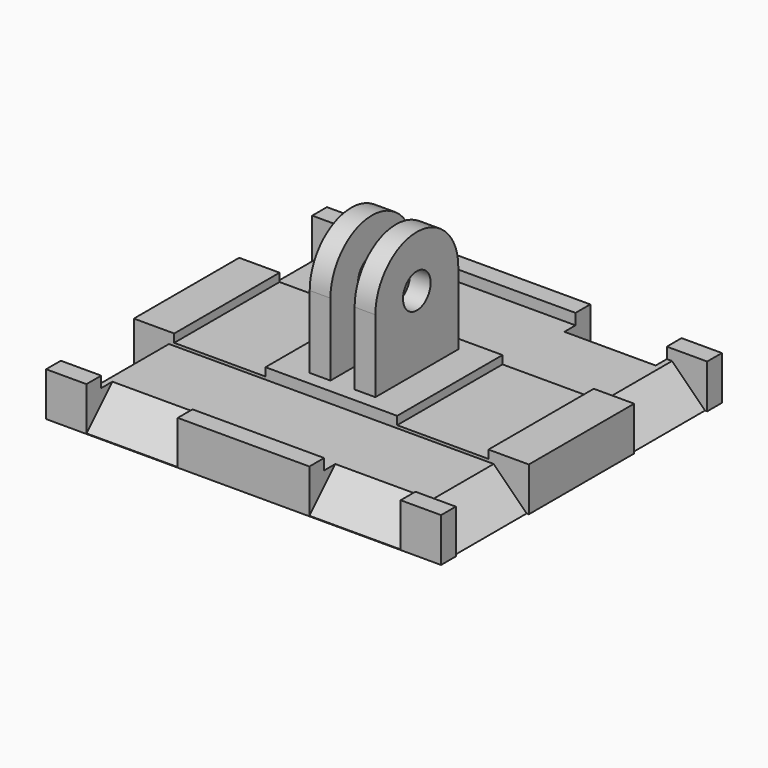
from build123d import *

# Parameters (mm, degrees)
F0_W         = 57.15
F0_H         = 50.8
F1_DEPTH     = 6.35
F2_W         = 13.208
F2_H         = 1.190625
F3_DEPTH     = 50.801
F4_SIZE      = 5.08
F5_W         = 3
F5_H         = 15
F6_DEPTH     = 18
F8_D         = 5
F9_W         = 13.208
F9_H         = 1.5875
F10_DEPTH    = 57.151
F11_T1_DEPTH = 13.208
F11_T3_DEPTH = 13.208
F13_DEPTH    = 33.326


# Not quite as in the source:
# - a fillet or chamfer that OpenCascade refuses, or shapes differently, is made with other operations: its cross-section is extruded or revolved along the edge and cut away or added


with BuildPart() as f1:
    # F0 (on Top) → F1 (new body)
    with BuildSketch(Plane.XY):
        Rectangle(F0_W, F0_H)
    extrude(amount=F1_DEPTH)

    # F2 (on face) → F3 (cut, through all)
    with BuildSketch(Plane.XZ.offset(25.4)):
        with Locations((-16.129, 5.7546875)):
            Rectangle(F2_W, F2_H)
        with Locations((16.129, 5.7546875)):
            Rectangle(F2_W, F2_H)
    extrude(amount=-F3_DEPTH, mode=Mode.SUBTRACT)

    # F4
    f4_edges = [f1.edges().sort_by_distance(p)[0] for p in [
        (-16.129, -25.4, 5.159375),
        (16.129, -25.4, 5.159375),
        (-16.129, 25.4, 5.159375),
        (16.129, 25.4, 5.159375),
    ]]
    chamfer(f4_edges, length=F4_SIZE)

    # F5 (on face) → F6 (join)
    with BuildSketch(Plane.XY.offset(6.35)):
        with Locations((-3.25, 0)):
            Rectangle(F5_W, F5_H)
        with Locations((3.25, 0)):
            Rectangle(F5_W, F5_H)
    extrude(amount=F6_DEPTH)

    # F8 (through all)
    with Locations(Plane.YZ.offset(4.75)):
        with Locations((0, 16.85)):
            Hole(F8_D / 2)

    # F9 (on face) → F10 (cut, through all)
    with BuildSketch(Plane.YZ.offset(28.575)):
        with Locations((-16.129, 5.55625)):
            Rectangle(F9_W, F9_H)
        with Locations((16.129, 5.55625)):
            Rectangle(F9_W, F9_H)
    extrude(amount=-F10_DEPTH, mode=Mode.SUBTRACT)

    # F11: chamfer of 5.08 on 4 edges, made by hand

    # F11_s2 → F11_t1 (cut)
    with BuildSketch(Plane.XZ.offset(-22.733)):
        Polygon((28.575, -0.3175), (23.495, 4.7625), (28.575, 4.7625), align=None)
        Polygon((-28.575, -0.3175), (-23.495, 4.7625), (-28.575, 4.7625), align=None)
    extrude(amount=F11_T1_DEPTH, mode=Mode.SUBTRACT)

    # F11_s4 → F11_t3 (cut)
    with BuildSketch(Plane.XZ.offset(9.525)):
        Polygon((28.575, -0.3175), (23.495, 4.7625), (28.575, 4.7625), align=None)
        Polygon((-28.575, -0.3175), (-23.495, 4.7625), (-28.575, 4.7625), align=None)
    extrude(amount=F11_T3_DEPTH, mode=Mode.SUBTRACT)

    # F12 (on face) → F13 (cut, through all)
    with BuildSketch(Plane(origin=(-4.75, 0, 0), x_dir=(0, -1, 0), z_dir=(-1, 0, 0))):
        with BuildLine():
            Line((-7.5, 24.35), (-7.5, 16.85))
            ThreePointArc((-7.5, 16.85), (-5.3033008589, 22.1533008589), (0, 24.35))
            Line((0, 24.35), (-7.5, 24.35))
        make_face()
        with BuildLine():
            Line((7.5, 24.35), (0, 24.35))
            ThreePointArc((0, 24.35), (5.3033008589, 22.1533008589), (7.5, 16.85))
            Line((7.5, 16.85), (7.5, 24.35))
        make_face()
    extrude(amount=-F13_DEPTH, mode=Mode.SUBTRACT)


solid = f1.part
